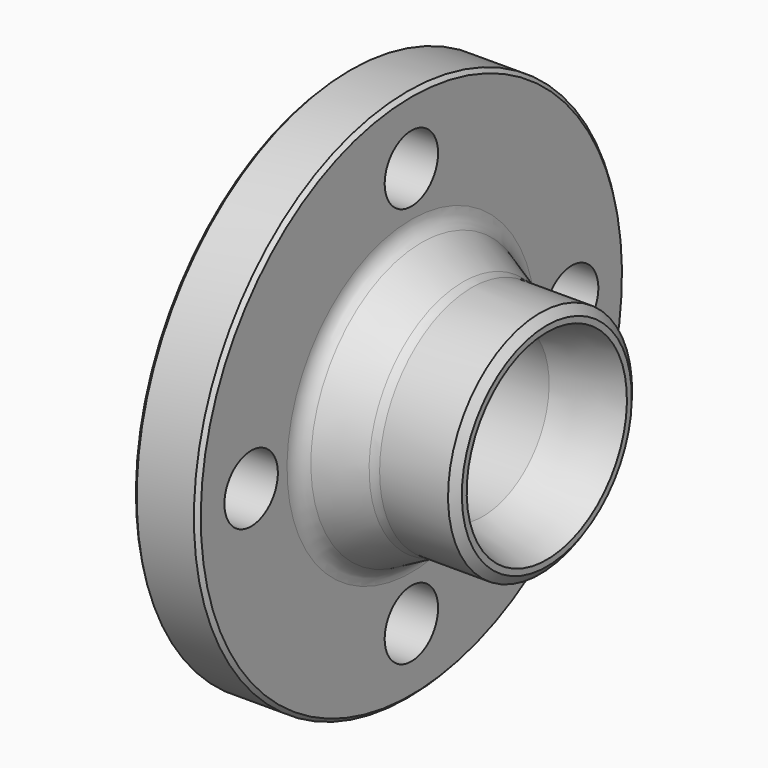
from build123d import *

# Parameters (mm, degrees)
F2_SIZE  = 1
F4_R     = 5
F5_R     = 8.75
F6_DEPTH = 52.501


# Not quite as in the source:
# - two fillets or chamfers of one size are made in one step


with BuildPart() as f1:
    # F0 (on Front) → F1 (revolve)
    with BuildSketch(Plane.XZ):
        Polygon((-3.5, 21.75), (35.7057713659, 21.75), (52.5, 26.25), (52.5, 27.84), (50.7274746578, 30.15), (31.5788313746, 30.15), (17, 37.7090089023), (17, 70), (0, 70), (0, 38.7), (6, 38.7), (6, 31.5), (0, 31.5), (0, 28), (-3.5, 28), align=None)
    revolve(axis=Axis((44.485598996, 0, 0), (1, 0, 0)))

    # F2
    f2_edges = [f1.edges().sort_by_distance(p)[0] for p in [
        (17, 0, -70),
        (0, 0, -70),
        (0, 0, -31.5),
        (0, 0, -28),
    ]]
    chamfer(f2_edges, length=F2_SIZE)

    # F4
    f4_edges = [f1.edges().sort_by_distance(p)[0] for p in [
        (17, 0, -37.709009),
        (31.578831, 0, -30.15),
    ]]
    fillet(f4_edges, radius=F4_R)

    # F5 (on face) → F6 (cut, through all)
    with BuildSketch(Plane(origin=(0, 0, 0), x_dir=(0, -1, 0), z_dir=(-1, 0, 0))):
        with Locations((0, 52.5)):
            Circle(F5_R)
        with Locations((-52.5, 0)):
            Circle(F5_R)
        with Locations((52.5, 0)):
            Circle(F5_R)
        with Locations((0, -52.5)):
            Circle(F5_R)
    extrude(amount=-F6_DEPTH, mode=Mode.SUBTRACT)


solid = f1.part
